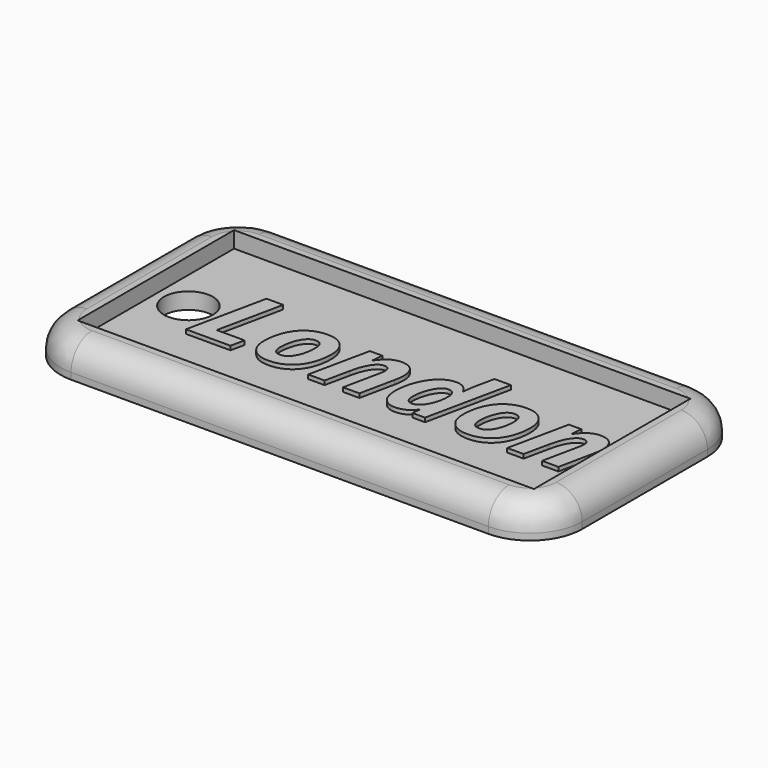
from build123d import *

# Parameters (mm, degrees)
F0_W         = 44.45
F0_H         = 19.05
F0_R         = 2.38125
F1_DEPTH     = 1.5875
F0_W_2       = 50.8
F0_H_2       = 25.4
F2_DEPTH     = 3.175
F3_R         = 5.08
F4_T1_DEPTH  = 40.64
F4_T3_DEPTH  = 15.24
F4_T6_ANGLE  = 90
F4_T8_ANGLE  = 90
F4_T10_ANGLE = 90
F4_T12_ANGLE = 90
F5_TEXT_SIZE = 10.8716393954
F6_DEPTH     = 0.396875


# Not quite as in the source:
# - a fillet or chamfer that OpenCascade refuses, or shapes differently, is made with other operations: its cross-section is extruded or revolved along the edge and cut away or added
# - Text() gives the source's letters only with a copy of the font that has no kerning and outlines rounded to 1/6400 em; it was checked with that copy


with BuildPart() as f1:
    # F0 (on Top) → F1 (new body)
    with BuildSketch(Plane.XY):
        with Locations((25.4, 12.7)):
            Rectangle(F0_W, F0_H)
        with Locations((6.35, 12.7)):
            Circle(F0_R, mode=Mode.SUBTRACT)
    extrude(amount=F1_DEPTH)

    # F0 (on Top) → F2 (join)
    with BuildSketch(Plane.XY):
        with Locations((25.4, 12.7)):
            Rectangle(F0_W_2, F0_H_2)
        with Locations((25.4, 12.7)):
            Rectangle(F0_W, F0_H, mode=Mode.SUBTRACT)
    extrude(amount=F2_DEPTH)

    # F3
    f3_edges = [f1.edges().sort_by_distance(p)[0] for p in [
        (50.8, 0, 1.5875),
        (0, 0, 1.5875),
        (0, 25.4, 1.5875),
        (50.8, 25.4, 1.5875),
    ]]
    fillet(f3_edges, radius=F3_R)

    # F4: fillet of radius 2.54 on 8 edges, made by hand

    # F4_s2 → F4_t1 (cut)
    with BuildSketch(Plane.YZ.offset(5.08)):
        with BuildLine():
            ThreePointArc((25.4, 0.635), (24.6560512242, 2.4310512242), (22.86, 3.175))
            Line((22.86, 3.175), (25.4, 3.175))
            Line((25.4, 3.175), (25.4, 0.635))
        make_face()
        with BuildLine():
            ThreePointArc((0, 0.635), (0.7439487758, 2.4310512242), (2.54, 3.175))
            Line((2.54, 3.175), (0, 3.175))
            Line((0, 3.175), (0, 0.635))
        make_face()
    extrude(amount=F4_T1_DEPTH, mode=Mode.SUBTRACT)

    # F4_s4 → F4_t3 (cut)
    with BuildSketch(Plane.XZ.offset(-20.32)):
        with BuildLine():
            ThreePointArc((0, 0.635), (0.7439487758, 2.4310512242), (2.54, 3.175))
            Line((2.54, 3.175), (0, 3.175))
            Line((0, 3.175), (0, 0.635))
        make_face()
        with BuildLine():
            ThreePointArc((50.8, 0.635), (50.0560512242, 2.4310512242), (48.26, 3.175))
            Line((48.26, 3.175), (50.8, 3.175))
            Line((50.8, 3.175), (50.8, 0.635))
        make_face()
    extrude(amount=F4_T3_DEPTH, mode=Mode.SUBTRACT)

    # F4_s5 → F4_t6 (revolve, cut)
    with BuildSketch(Plane.XZ.offset(-20.32)):
        with BuildLine():
            ThreePointArc((0, 0.635), (0.7439487758, 2.4310512242), (2.54, 3.175))
            Line((2.54, 3.175), (0, 3.175))
            Line((0, 3.175), (0, 0.635))
        make_face()
    revolve(axis=Axis((5.08, 20.32, 3.175), (0, 0, -1)), revolution_arc=F4_T6_ANGLE, mode=Mode.SUBTRACT)

    # F4_s7 → F4_t8 (revolve, cut)
    with BuildSketch(Plane.XZ.offset(-5.08)):
        with BuildLine():
            ThreePointArc((0, 0.635), (0.7439487758, 2.4310512242), (2.54, 3.175))
            Line((2.54, 3.175), (0, 3.175))
            Line((0, 3.175), (0, 0.635))
        make_face()
    revolve(axis=Axis((5.08, 5.08, 3.175), (0, 0, 1)), revolution_arc=F4_T8_ANGLE, mode=Mode.SUBTRACT)

    # F4_s9 → F4_t10 (revolve, cut)
    with BuildSketch(Plane.XZ.offset(-20.32)):
        with BuildLine():
            ThreePointArc((50.8, 0.635), (50.0560512242, 2.4310512242), (48.26, 3.175))
            Line((48.26, 3.175), (50.8, 3.175))
            Line((50.8, 3.175), (50.8, 0.635))
        make_face()
    revolve(axis=Axis((45.72, 20.32, 3.175), (0, 0, 1)), revolution_arc=F4_T10_ANGLE, mode=Mode.SUBTRACT)

    # F4_s11 → F4_t12 (revolve, cut)
    with BuildSketch(Plane.YZ.offset(45.72)):
        with BuildLine():
            ThreePointArc((0, 0.635), (0.7439487758, 2.4310512242), (2.54, 3.175))
            Line((2.54, 3.175), (0, 3.175))
            Line((0, 3.175), (0, 0.635))
        make_face()
    revolve(axis=Axis((45.72, 5.08, 3.175), (0, 0, 1)), revolution_arc=F4_T12_ANGLE, mode=Mode.SUBTRACT)

    # F5 (on face) → F6 (join)
    with BuildSketch(Plane.XY.offset(1.5875)):
        with Locations((8.8096788613, 8.969414768)):
            Text('London', F5_TEXT_SIZE, font='Open Sans', font_style=FontStyle.BOLDITALIC, text_align=(TextAlign.LEFT, TextAlign.BOTTOM))
    extrude(amount=F6_DEPTH)


solid = f1.part
